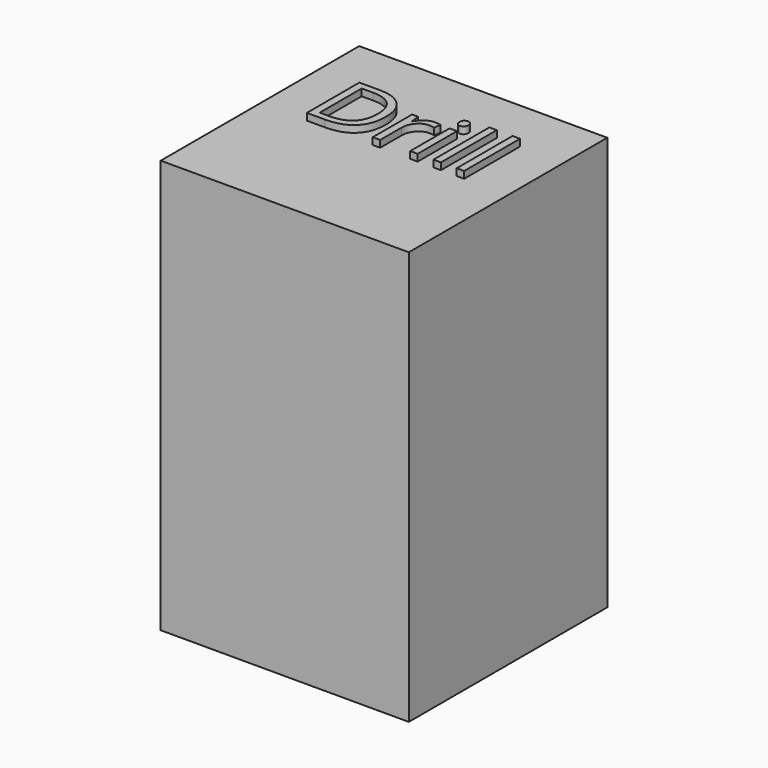
from build123d import *

# Parameters (mm, degrees)
F0_W         = 914.4
F0_H         = 914.4
F1_DEPTH     = 1524
F2_TEXT_SIZE = 338.6384467961
F3_DEPTH     = 25.4


# Not quite as in the source:
# - Text() gives the source's letters only with a copy of the font that has no kerning and outlines rounded to 1/6400 em; it was checked with that copy


with BuildPart() as f1:
    # F0 (on Top) → F1 (new body)
    with BuildSketch(Plane.XY):
        Rectangle(F0_W, F0_H)
    extrude(amount=F1_DEPTH)

    # F2 (on face) → F3 (join)
    with BuildSketch(Plane.XY.offset(1524)):
        with Locations((-317.5, 0)):
            Text('Drill', F2_TEXT_SIZE, font='Open Sans', text_align=(TextAlign.LEFT, TextAlign.BOTTOM))
    extrude(amount=F3_DEPTH)


solid = f1.part
